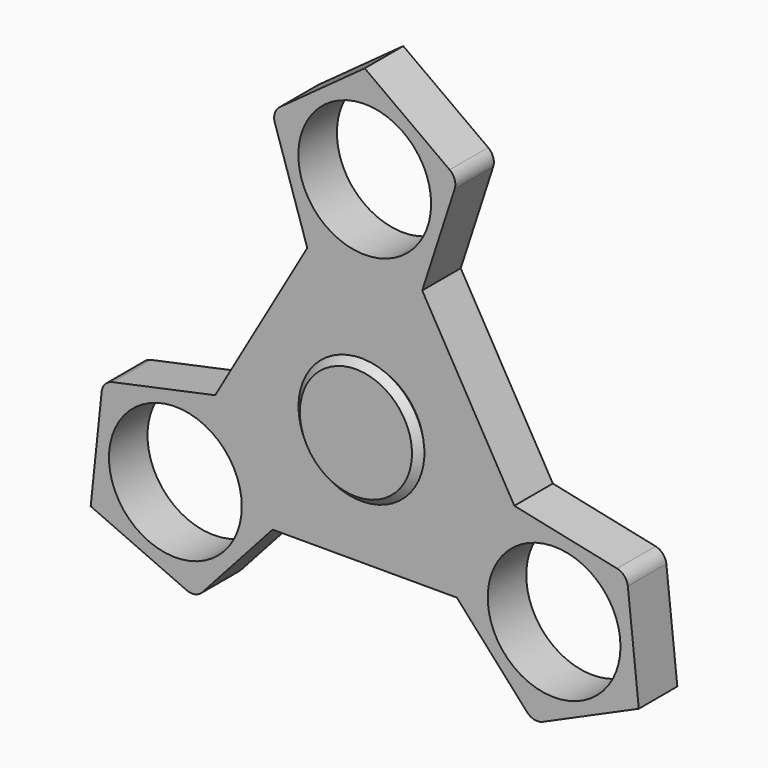
from build123d import *

# Parameters (mm, degrees)
F0_R     = 9.65
F0_R_2   = 8.6
F1_DEPTH = 7
F2_R     = 2
F3_R     = 2
F6_SIZE  = 0.99999
F7_W     = 1.8
F7_H     = 5.9
F9_SIZE  = 0.99999


# Not quite as in the source:
# - a fillet or chamfer is up to 0.001 mm smaller than in the source, because OpenCascade refuses the exact size


with BuildPart() as f1:
    # F0 (on Front) → F1 (new body)
    with BuildSketch(Plane.XZ):
        Polygon((21.7451338694, -2.9067598383), (8.3552390721, 20.2852182588), (-8.3552390721, 20.2852182588), (-21.7451338694, -2.9067598383), (-38.0904479732, -6.3810636036), (-39.8371685741, -23), (-24.5713871705, -29.7967637845), (-13.3898947974, -17.3784584205), (13.3898947974, -17.3784584205), (24.5713871705, -29.7967637845), (39.8371685741, -23), (38.0904479732, -6.3810636036), align=None)
        with Locations((-27.5268064769, -15.8926091294)):
            Circle(F0_R, mode=Mode.SUBTRACT)
        with Locations((27.5268064769, -15.8926091294)):
            Circle(F0_R, mode=Mode.SUBTRACT)
        with BuildLine():
            Line((-13.9218488041, 8.0377831547), (-13.0164978485, 9.3043421992))
            ThreePointArc((-13.0164978485, 9.3043421992), (0, 16), (13.0164978485, 9.3043421992))
            Line((13.0164978485, 9.3043421992), (13.9218488041, 8.0377831547))
            Line((13.9218488041, 8.0377831547), (14.5660456343, 6.6204467055))
            ThreePointArc((14.5660456343, 6.6204467055), (15.6374027599, 3.3869802075), (16, 0))
            ThreePointArc((16, 0), (11.8488979355, -10.7519122817), (1.5495477858, -15.9247889047))
            Line((1.5495477858, -15.9247889047), (0, -16.0755663093))
            Line((0, -16.0755663093), (-1.5495477858, -15.9247889047))
            ThreePointArc((-1.5495477858, -15.9247889047), (-13.8564064606, -8), (-14.5660456343, 6.6204467055))
            Line((-14.5660456343, 6.6204467055), (-13.9218488041, 8.0377831547))
        make_face(mode=Mode.SUBTRACT)
        with BuildLine():
            ThreePointArc((13.0164978485, 9.3043421992), (0, 16), (-13.0164978485, 9.3043421992))
            ThreePointArc((-13.0164978485, 9.3043421992), (-13.8564064606, 8), (-14.5660456343, 6.6204467055))
            ThreePointArc((-14.5660456343, 6.6204467055), (-13.8564064606, -8), (-1.5495477858, -15.9247889047))
            ThreePointArc((-1.5495477858, -15.9247889047), (0, -16), (1.5495477858, -15.9247889047))
            ThreePointArc((1.5495477858, -15.9247889047), (11.8488979355, -10.7519122817), (16, 0))
            ThreePointArc((16, 0), (15.6374027599, 3.3869802075), (14.5660456343, 6.6204467055))
            ThreePointArc((14.5660456343, 6.6204467055), (13.8564064606, 8), (13.0164978485, 9.3043421992))
        make_face()
        Circle(F0_R_2, mode=Mode.SUBTRACT)
        Polygon((8.3552390721, 20.2852182588), (13.5190608027, 36.1778273881), (0, 46), (-13.5190608027, 36.1778273881), (-8.3552390721, 20.2852182588), align=None)
        with Locations((0, 31.7852182588)):
            Circle(F0_R, mode=Mode.SUBTRACT)
        with BuildLine():
            ThreePointArc((-14.5660456343, 6.6204467055), (-13.8564064606, 8), (-13.0164978485, 9.3043421992))
            Line((-13.0164978485, 9.3043421992), (-13.9218488041, 8.0377831547))
            Line((-13.9218488041, 8.0377831547), (-14.5660456343, 6.6204467055))
        make_face()
        with BuildLine():
            Line((13.9218488041, 8.0377831547), (13.0164978485, 9.3043421992))
            ThreePointArc((13.0164978485, 9.3043421992), (13.8564064606, 8), (14.5660456343, 6.6204467055))
            Line((14.5660456343, 6.6204467055), (13.9218488041, 8.0377831547))
        make_face()
        with BuildLine():
            ThreePointArc((1.5495477858, -15.9247889047), (0, -16), (-1.5495477858, -15.9247889047))
            Line((-1.5495477858, -15.9247889047), (0, -16.0755663093))
            Line((0, -16.0755663093), (1.5495477858, -15.9247889047))
        make_face()
    extrude(amount=F1_DEPTH)

    # F2
    f2_edges = [f1.edges().sort_by_distance(p)[0] for p in [
        (-13.519061, -3.5, 36.177827),
    ]]
    fillet(f2_edges, radius=F2_R)

    # F3
    f3_edges = [f1.edges().sort_by_distance(p)[0] for p in [
        (13.519061, -3.5, 36.177827),
        (38.090448, -3.5, -6.381064),
        (24.571387, -3.5, -29.796764),
        (-38.090448, -3.5, -6.381064),
        (-24.571387, -3.5, -29.796764),
    ]]
    fillet(f3_edges, radius=F3_R)


with BuildPart() as f5:
    # F4 (on Top) → F5 (revolve)
    with BuildSketch(Plane.XY):
        Polygon((-2.9, 0.5), (-2.9, 0), (-2.9, -7), (-1.9, -7), (-1.9, -1), (0, -1), (0, 1.5), (-9.15, 1.5), (-9.15, 0.5), align=None)
    revolve(axis=Axis((0, 0.25, 0), (0, 1, 0)))

    # F6 (size 1 in the source; OpenCascade refuses exactly that, so slightly less here)
    f6_edges = [f5.edges().sort_by_distance(p)[0] for p in [
        (9.15, 1.5, 0),
    ]]
    chamfer(f6_edges, length=F6_SIZE)


with BuildPart() as f8:
    # F7 (on Top) → F8 (revolve)
    with BuildSketch(Plane.XY):
        Polygon((0, -8.6), (0, -7), (-1.8, -7), (-1.8, -7.6), (-9.15, -7.6), (-9.15, -8.6), align=None)
        with Locations((-0.9, -4.05)):
            Rectangle(F7_W, F7_H)
    revolve(axis=Axis((0, -4.85, 0), (0, -1, 0)))

    # F9 (size 1 in the source; OpenCascade refuses exactly that, so slightly less here)
    f9_edges = [f8.edges().sort_by_distance(p)[0] for p in [
        (9.15, -8.6, 0),
    ]]
    chamfer(f9_edges, length=F9_SIZE)


solid = Compound([f1.part, f5.part, f8.part])
